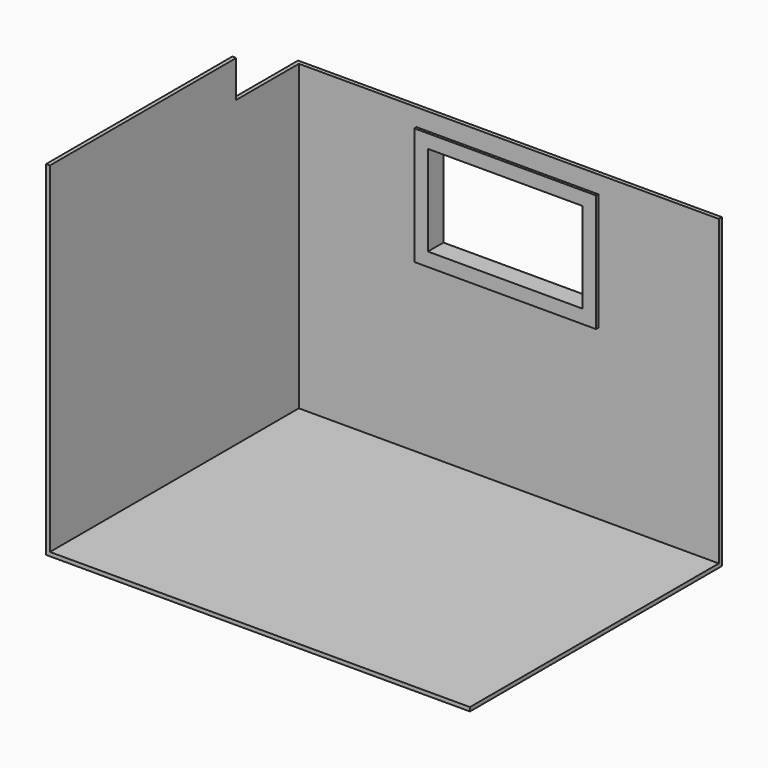
from build123d import *

# Parameters (mm, degrees)
F0_W      = 2743.2
F0_H      = 2032
F1_DEPTH  = 25.4
F2_W      = 25.4
F2_H      = 2032
F3_DEPTH  = 2006.6
F4_W      = 1187.45
F4_H      = 768.35
F4_W_2    = 1009.65
F4_H_2    = 590.55
F5_DEPTH  = 17.78
F6_DEPTH  = 25.4
F7_W      = 1047.75
F7_H      = 628.65
F7_W_2    = 1009.65
F7_H_2    = 590.55
F8_DEPTH  = 83.82
F9_W      = 25.4
F9_H      = 1520.825
F10_DEPTH = 241.3


with BuildPart() as f1:
    # F0 (on Top) → F1 (new body)
    with BuildSketch(Plane.XY):
        with Locations((1371.6, -1016)):
            Rectangle(F0_W, F0_H)
    extrude(amount=F1_DEPTH)

    # F2 (on Top) → F3 (join)
    with BuildSketch(Plane.XY):
        with Locations((-12.7, -1016)):
            Rectangle(F2_W, F2_H)
        Polygon((-25.4, 0), (0, 0), (2743.2, 0), (2743.2, 25.4), (-25.4, 25.4), align=None)
    extrude(amount=F3_DEPTH)

    # F4 (on face) → F5 (join)
    with BuildSketch(Plane.XZ):
        with Locations((1362.075, 1508.125)):
            Rectangle(F4_W, F4_H)
        with Locations((1362.075, 1508.125)):
            Rectangle(F4_W_2, F4_H_2, mode=Mode.SUBTRACT)
    extrude(amount=F5_DEPTH)

    # F6 (cut): a face of the model
    f6_faces = [f1.faces().sort_by_distance(p)[0] for p in [
        (1362.075, 0, 1508.125),
    ]]
    extrude(f6_faces, amount=-F6_DEPTH, mode=Mode.SUBTRACT)

    # F7 (on face) → F8 (join)
    with BuildSketch(Plane(origin=(0, 25.4, 0), x_dir=(-1, 0, 0), z_dir=(0, 1, 0))):
        with Locations((-1362.075, 1508.125)):
            Rectangle(F7_W, F7_H)
        with Locations((-1362.075, 1508.125)):
            Rectangle(F7_W_2, F7_H_2, mode=Mode.SUBTRACT)
    extrude(amount=F8_DEPTH)

    # F9 (on face) → F10 (join)
    with BuildSketch(Plane.XY.offset(2006.6)):
        with Locations((-12.7, -1271.5875)):
            Rectangle(F9_W, F9_H)
    extrude(amount=F10_DEPTH)


solid = f1.part
